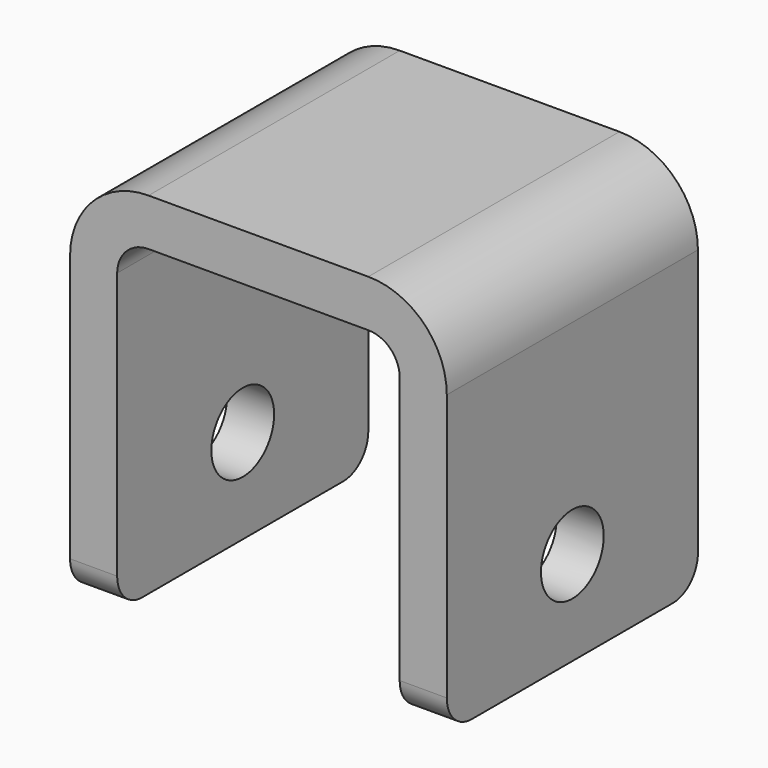
from build123d import *

# Parameters (mm, degrees)
F0_W     = 76.2
F0_H     = 76.2
F1_DEPTH = 63.5
F2_T     = -9.525
F3_R     = 6.35
F4_R     = 15.875
F5_R     = 7.9375
F6_DEPTH = 76.201
F7_R     = 6.35


with BuildPart() as f1:
    # F0 (on Front) → F1 (new body)
    with BuildSketch(Plane.XZ):
        with Locations((7.4331681192, 38.1)):
            Rectangle(F0_W, F0_H)
    extrude(amount=-F1_DEPTH)

    # F2
    f2_openings = [f1.faces().sort_by_distance(p)[0] for p in [
        (7.433168, 0, 38.1),
        (7.433168, 31.75, 0),
        (7.433168, 63.5, 38.1),
    ]]
    offset(amount=F2_T, openings=f2_openings)

    # F3
    f3_edges = [f1.edges().sort_by_distance(p)[0] for p in [
        (-21.141832, 31.75, 66.675),
        (36.008168, 31.75, 66.675),
    ]]
    fillet(f3_edges, radius=F3_R)

    # F4
    f4_edges = [f1.edges().sort_by_distance(p)[0] for p in [
        (-30.666832, 31.75, 76.2),
        (45.533168, 31.75, 76.2),
    ]]
    fillet(f4_edges, radius=F4_R)

    # F5 (on face) → F6 (cut, through all)
    with BuildSketch(Plane.YZ.offset(45.5331681192)):
        with Locations((31.75, 19.05)):
            Circle(F5_R)
    extrude(amount=-F6_DEPTH, mode=Mode.SUBTRACT)

    # F7
    f7_edges = [f1.edges().sort_by_distance(p)[0] for p in [
        (-25.904332, 0, 0),
        (40.770668, 0, 0),
        (-25.904332, 63.5, 0),
        (40.770668, 63.5, 0),
    ]]
    fillet(f7_edges, radius=F7_R)


solid = f1.part
